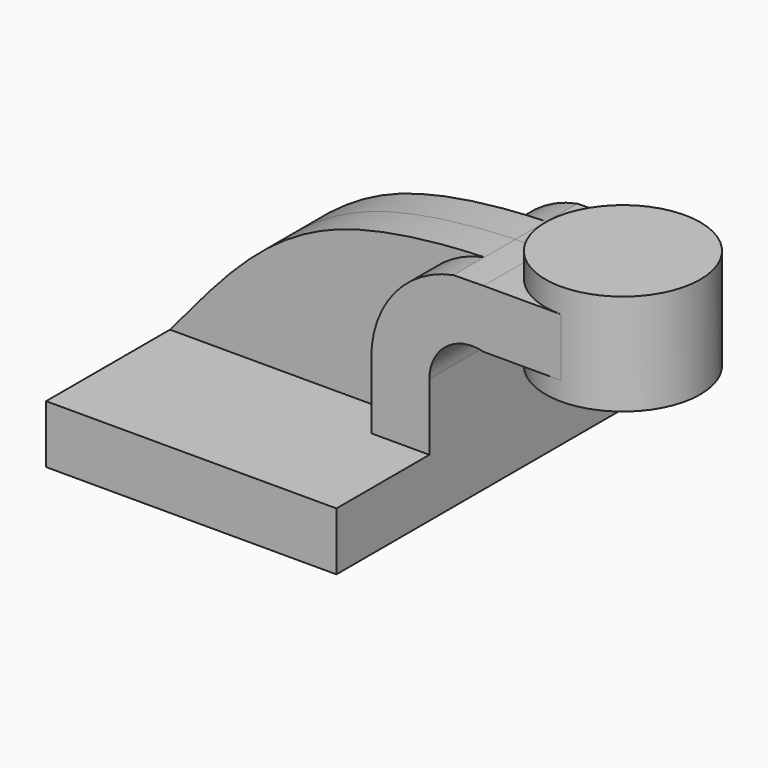
from build123d import *

# Parameters (mm, degrees)
F1_DEPTH = 63.5
F2_DEPTH = 12.7
F0_W     = 25.4
F0_H     = 19.0624117216
F3_DEPTH = 25.4


# Not quite as in the source:
# - a feature names something its author has since deleted; it is built from what else it names


with BuildPart() as f1:
    # F0 (on Front) → F1 (new body, symmetric)
    with BuildSketch(Plane.XZ):
        Polygon((47.625, -9.525), (47.625, 9.525), (28.575, 9.525), (-47.625, 9.525), (-47.625, -9.525), align=None)
    extrude(amount=F1_DEPTH, both=True)

    # F0 (on Front) → F2 (join, symmetric)
    with BuildSketch(Plane.XZ):
        with BuildLine():
            Line((-47.625, 9.525), (28.575, 9.525))
            Line((28.575, 9.525), (28.575, 31.3774505112))
            ThreePointArc((28.575, 31.3774505112), (36.1870844323, 52.5292330788), (55.5320502217, 63.9797367269))
            add(Edge.make_bspline(
                [(-47.625, 9.525), (-32.001836586, 27.9945600123), (-8.2663538638, 59.5795130057), (42.691262939, 63.5782592588), (55.5320502217, 63.9797367269)],
                knots=[0, 0, 0, 0, 0.463039199, 0.7597377555, 0.7597377555, 0.7597377555, 0.7597377555], degree=3))
        make_face()
    extrude(amount=F2_DEPTH, both=True)

    # F0 (on Front) → F3 (join, symmetric)
    with BuildSketch(Plane.XZ):
        with BuildLine():
            Line((28.575, 9.525), (47.625, 9.525))
            Line((47.625, 9.525), (47.625, 31.3774505112))
            ThreePointArc((47.625, 31.3774505112), (53.1477549989, 42.5899481953), (65.4029340449, 45.0458622098))
            Line((65.4029340449, 45.0458622098), (65.4029340449, 64.1082739314))
            add(Edge.make_bspline(
                [(55.5320502217, 63.9797367269), (59.6889735266, 64.1097062534), (63.1060550499, 64.1180929217), (65.4029340449, 64.1082739314)],
                knots=[0.7597377555, 0.7597377555, 0.7597377555, 0.7597377555, 0.8557874071, 0.8557874071, 0.8557874071, 0.8557874071], degree=3))
            ThreePointArc((55.5320502217, 63.9797367269), (36.1870844323, 52.5292330788), (28.575, 31.3774505112))
            Line((28.575, 31.3774505112), (28.575, 9.525))
        make_face()
        with Locations((78.1029340449, 54.5770680706)):
            Rectangle(F0_W, F0_H)
    extrude(amount=F3_DEPTH, both=True)

    # F0 (on Front) → F4 (revolve)
    with BuildSketch(Plane.XZ):
        Polygon((90.8029340449, 64.1082739314), (90.8029340449, 45.0458622098), (90.8029340449, 38.931951193), (116.2029340449, 38.931951193), (116.2029340449, 72.13054624), (90.8029340449, 72.13054624), align=None)
    revolve(axis=Axis((90.8029340449, 0, 55.5312487165), (0, 0, -1)))


solid = f1.part
